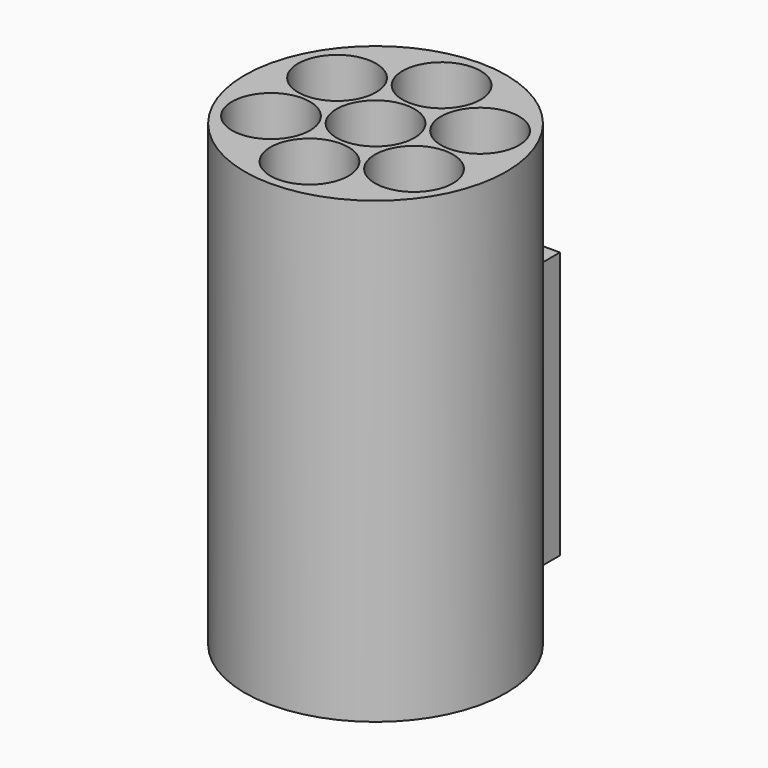
from build123d import *

# Parameters (mm, degrees)
F2_R         = 1.425
F3_DEPTH     = 5
F8_TEXT_SIZE = 4.0725106373
F9_DEPTH     = 0.35
F1_R         = 0.425
F10_DEPTH    = 5.001


# Not quite as in the source:
# - Text() gives the source's letters only with a copy of the font that has no kerning and outlines rounded to 1/6400 em; it was checked with that copy


with BuildPart() as f3:
    # F2 (on Top) → F3 (new body)
    with BuildSketch(Plane.XY):
        Circle(F2_R)
    extrude(amount=F3_DEPTH)

    # F8 (on face) → F9 (join)
    with BuildSketch(Plane(origin=(0, 1.225, 0), x_dir=(-1, 0, 0), z_dir=(0, 1, 0))):
        with Locations((-1.1491243131, 0.4582579713)):
            Text('II', F8_TEXT_SIZE, font='Open Sans', text_align=(TextAlign.LEFT, TextAlign.BOTTOM))
        with Locations((-0.6036871637, 0.4582579713)):
            Text('I', F8_TEXT_SIZE, font='Open Sans', text_align=(TextAlign.LEFT, TextAlign.BOTTOM))
    extrude(amount=F9_DEPTH)

    # F1 (on Top) → F10 (cut, through all)
    with BuildSketch(Plane.XY):
        Circle(F1_R)
        with Locations((0, 0.9)):
            Circle(F1_R)
        with Locations((0.7794228634, 0.45)):
            Circle(F1_R)
        with Locations((0.7794228634, -0.45)):
            Circle(F1_R)
        with Locations((0, -0.9)):
            Circle(F1_R)
        with Locations((-0.7794228634, -0.45)):
            Circle(F1_R)
        with Locations((-0.7794228634, 0.45)):
            Circle(F1_R)
    extrude(amount=F10_DEPTH, mode=Mode.SUBTRACT)


solid = f3.part
